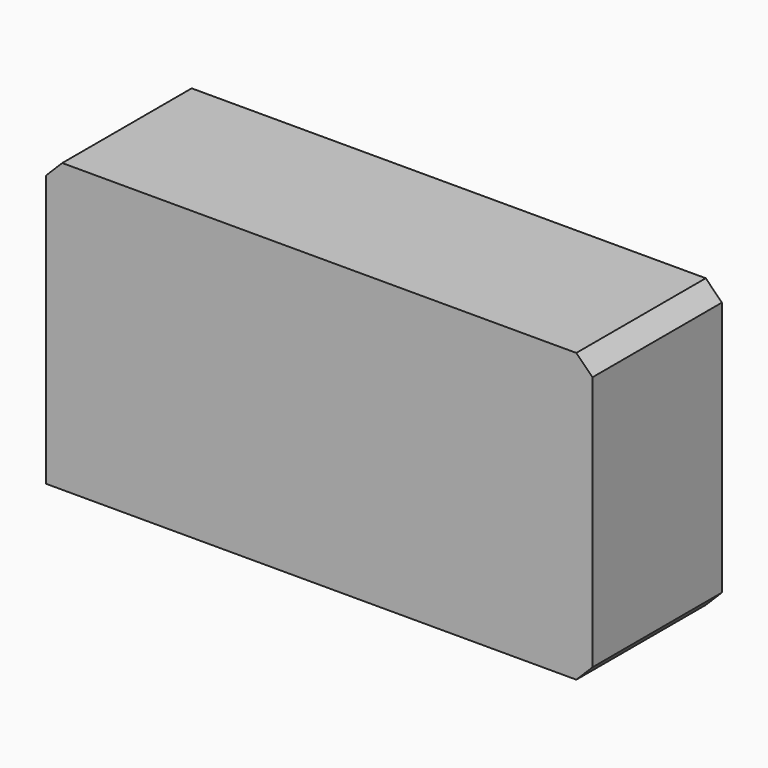
from build123d import *

# Parameters (mm, degrees)
F0_W     = 171.5900823474
F0_H     = 90.3337560594
F1_DEPTH = 50.8
F3_SIZE  = 5.08


# Not quite as in the source:
# - a feature names something its author has since deleted; it is built from what else it names


with BuildPart() as f1:
    # F0 (on Front) → F1 (new body)
    with BuildSketch(Plane.XZ):
        with Locations((9.5528103411, 11.7697473615)):
            Rectangle(F0_W, F0_H)
    extrude(amount=F1_DEPTH)

    # F3
    f3_edges = [f1.edges().sort_by_distance(p)[0] for p in [
        (-76.242231, -25.4, 56.936625),
        (95.347852, -25.4, 56.936625),
        (95.347852, -25.4, -33.397131),
    ]]
    chamfer(f3_edges, length=F3_SIZE)


solid = f1.part
